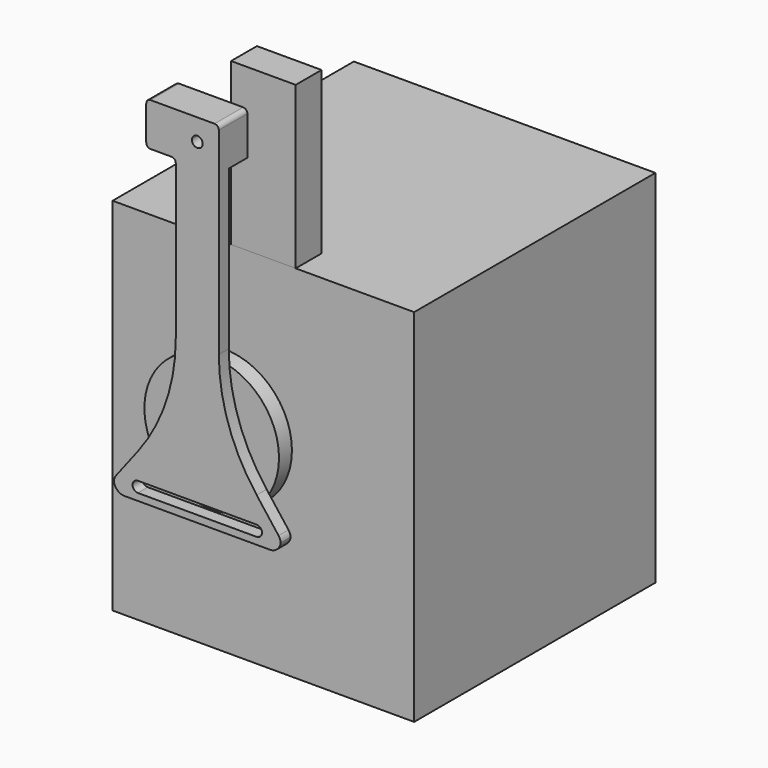
from build123d import *

# Parameters (mm, degrees)
F0_W         = 177.8
F0_H         = 177.8
F1_DEPTH     = 212.725
F2_W         = 38.1
F2_H         = 19.05
F3_DEPTH     = 95.25
F4_R         = 6.35
F5_DEPTH     = 38.1
F6_R         = 39.6875
F7_DEPTH     = 9.525
F9_R         = 1.9685
F10_DEPTH    = 3.302
F12_DEPTH    = 7.3152
F14_T1_DEPTH = 18.0928727189
F14_T3_DEPTH = 39.0652
F15_R        = 107.95
F16_R        = 3.175
F17_DEPTH    = 7.3152
F19_DEPTH    = 13.716
F20_W        = 42.799
F20_H        = 25.4
F20_R        = 3.175
F21_DEPTH    = 7.3152
F22_R        = 2.54


# Not quite as in the source:
# - a fillet or chamfer that OpenCascade refuses, or shapes differently, is made with other operations: its cross-section is extruded or revolved along the edge and cut away or added


with BuildPart() as f1:
    # F0 (on Top) → F1 (new body)
    with BuildSketch(Plane.XY):
        Rectangle(F0_W, F0_H)
    extrude(amount=F1_DEPTH)

    # F4 (on face) → F5 (join)
    with BuildSketch(Plane.XZ.offset(88.9)):
        with Locations((0, 136.525)):
            Circle(F4_R)
    extrude(amount=F5_DEPTH)


with BuildPart() as f3:
    # F2 (on face) → F3 (new body)
    with BuildSketch(Plane.XY.offset(212.725)):
        with Locations((0, -79.375)):
            Rectangle(F2_W, F2_H)
    extrude(amount=F3_DEPTH)


with BuildPart() as f7:
    # F6 (on face) → F7 (new body)
    with BuildSketch(Plane.XZ.offset(127)):
        with Locations((0, 136.525)):
            Circle(F6_R)
    extrude(amount=-F7_DEPTH)

    # F8: cut F1
    add(f1.part, mode=Mode.SUBTRACT)

    # F9 (on face) → F10 (join)
    with BuildSketch(Plane.XZ.offset(127)):
        with Locations((0, 101.525)):
            Circle(F9_R)
    extrude(amount=F10_DEPTH)


with BuildPart() as f12:
    # F11 (on face) → F12 (new body)
    with BuildSketch(Plane.XZ.offset(130.302)):
        Polygon((-49.2125, 94.2225), (49.2125, 94.2225), (49.2125, 101.525), (12.7, 149.1090164259), (12.7, 304.725), (-12.7, 304.725), (-12.7, 149.1090164259), (-49.2125, 101.525), align=None)
        with BuildLine():
            Line((-35, 104.7), (35, 104.7))
            ThreePointArc((35, 104.7), (38.175, 101.525), (35, 98.35))
            Line((35, 98.35), (-35, 98.35))
            ThreePointArc((-35, 98.35), (-38.175, 101.525), (-35, 104.7))
        make_face(mode=Mode.SUBTRACT)
    extrude(amount=F12_DEPTH)

    # F14: fillet of radius 6.35 on 4 edges, made by hand

    # F14_s2 → F14_t1 (cut)
    with BuildSketch(Plane.XZ.offset(124.9131636405)):
        with BuildLine():
            ThreePointArc((-47.9002937108, 103.2351005304), (-48.8755063223, 101.4106060609), (-49.2125, 99.3694654562))
            Line((-49.2125, 99.3694654562), (-49.2125, 101.525))
            Line((-49.2125, 101.525), (-47.9002937108, 103.2351005304))
        make_face()
        with BuildLine():
            ThreePointArc((49.2125, 99.3694654562), (48.8755063223, 101.4106060609), (47.9002937108, 103.2351005304))
            Line((47.9002937108, 103.2351005304), (49.2125, 101.525))
            Line((49.2125, 101.525), (49.2125, 99.3694654562))
        make_face()
    extrude(amount=F14_T1_DEPTH, mode=Mode.SUBTRACT)

    # F14_s4 → F14_t3 (cut)
    with BuildSketch(Plane.XZ.offset(114.427)):
        with BuildLine():
            ThreePointArc((-49.2125, 100.5725), (-47.3526280605, 96.0823719395), (-42.8625, 94.2225))
            Line((-42.8625, 94.2225), (-49.2125, 94.2225))
            Line((-49.2125, 94.2225), (-49.2125, 100.5725))
        make_face()
        with BuildLine():
            ThreePointArc((42.8625, 94.2225), (47.3526280605, 96.0823719395), (49.2125, 100.5725))
            Line((49.2125, 100.5725), (49.2125, 94.2225))
            Line((49.2125, 94.2225), (42.8625, 94.2225))
        make_face()
    extrude(amount=F14_T3_DEPTH, mode=Mode.SUBTRACT)

    # F15
    f15_edges = [f12.edges().sort_by_distance(p)[0] for p in [
        (-12.7, -133.9596, 149.109016),
        (12.7, -133.9596, 149.109016),
    ]]
    fillet(f15_edges, radius=F15_R)

    # F16 (on face) → F17 (cut, through all)
    with BuildSketch(Plane.XZ.offset(137.6172)):
        with Locations((0, 292.025)):
            Circle(F16_R)
    extrude(amount=-F17_DEPTH, mode=Mode.SUBTRACT)

    # F18 (on face) → F19 (join)
    with BuildSketch(Plane(origin=(0, -130.302, 0), x_dir=(-1, 0, 0), z_dir=(0, 1, 0))):
        with BuildLine():
            Line((-6.4135, 299.645), (30.099, 299.645))
            Line((30.099, 299.645), (30.099, 304.725))
            Line((30.099, 304.725), (-12.7, 304.725))
            Line((-12.7, 304.725), (-12.7, 279.325))
            Line((-12.7, 279.325), (30.099, 279.325))
            Line((30.099, 279.325), (30.099, 284.405))
            Line((30.099, 284.405), (-6.4135, 284.405))
            ThreePointArc((-6.4135, 284.405), (-7.5360320151, 284.8699679849), (-8.001, 285.9925))
            Line((-8.001, 285.9925), (-8.001, 298.0575))
            ThreePointArc((-8.001, 298.0575), (-7.5360320151, 299.1800320151), (-6.4135, 299.645))
        make_face()
    extrude(amount=F19_DEPTH)

    # F20 (on face) → F21 (join, through all)
    with BuildSketch(Plane.XZ.offset(130.302)):
        with Locations((-8.6995, 292.025)):
            Rectangle(F20_W, F20_H)
        with Locations((0, 292.025)):
            Circle(F20_R, mode=Mode.SUBTRACT)
    extrude(amount=F21_DEPTH)

    # F22
    f22_edges = [f12.edges().sort_by_distance(p)[0] for p in [
        (-12.7, -133.9596, 279.325),
        (-30.099, -127.1016, 279.325),
        (-30.099, -127.1016, 304.725),
        (12.7, -127.1016, 304.725),
    ]]
    fillet(f22_edges, radius=F22_R)


solid = Compound([f1.part, f3.part, f7.part, f12.part])
